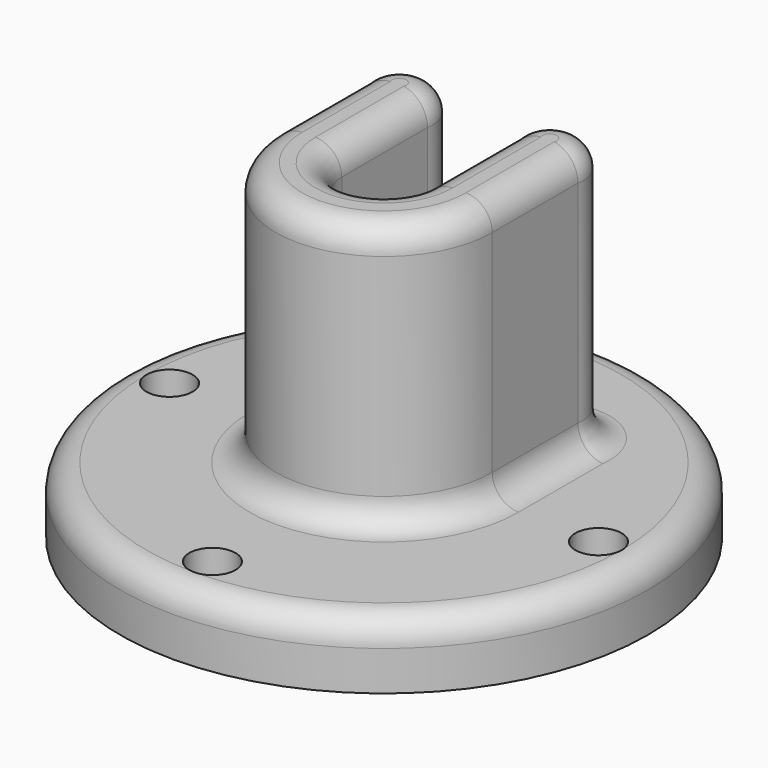
from build123d import *

# Parameters (mm, degrees)
F0_R     = 25.4
F0_R_2   = 2.2225
F1_DEPTH = 6.35
F3_DEPTH = 25.4
F5_R     = 2.54
F6_DEPTH = 25.4


# Not quite as in the source:
# - a feature of the source that left no trace in its solid (it failed there, or was rolled back) is left out


with BuildPart() as f1:
    # F0 (on Top) → F1 (new body)
    with BuildSketch(Plane.XY):
        Circle(F0_R)
        with Locations((0, -20.6375)):
            Circle(F0_R_2, mode=Mode.SUBTRACT)
        with Locations((-20.6375, 0)):
            Circle(F0_R_2, mode=Mode.SUBTRACT)
        with Locations((20.6375, 0)):
            Circle(F0_R_2, mode=Mode.SUBTRACT)
        with BuildLine():
            Line((-4.064, 10.31875), (-4.064, 0))
            ThreePointArc((-4.064, 0), (0, -4.064), (4.064, 0))
            Line((4.064, 0), (4.064, 10.31875))
            ThreePointArc((4.064, 10.31875), (7.239, 14.1114143812), (10.414, 10.31875))
            Line((10.414, 10.31875), (10.414, 0))
            ThreePointArc((10.414, 0), (0, -10.414), (-10.414, 0))
            Line((-10.414, 0), (-10.414, 10.31875))
            ThreePointArc((-10.414, 10.31875), (-7.239, 14.1114143812), (-4.064, 10.31875))
        make_face(mode=Mode.SUBTRACT)
        with Locations((0, 20.6375)):
            Circle(F0_R_2, mode=Mode.SUBTRACT)
        with BuildLine():
            ThreePointArc((4.064, 0), (0, -4.064), (-4.064, 0))
            Line((-4.064, 0), (-4.064, 10.31875))
            ThreePointArc((-4.064, 10.31875), (-7.239, 14.1114143812), (-10.414, 10.31875))
            Line((-10.414, 10.31875), (-10.414, 0))
            ThreePointArc((-10.414, 0), (0, -10.414), (10.414, 0))
            Line((10.414, 0), (10.414, 10.31875))
            ThreePointArc((10.414, 10.31875), (7.239, 14.1114143812), (4.064, 10.31875))
            Line((4.064, 10.31875), (4.064, 0))
        make_face()
        with Locations((0, -20.6375)):
            Circle(F0_R_2)
        with Locations((-20.6375, 0)):
            Circle(F0_R_2)
        with Locations((0, 20.6375)):
            Circle(F0_R_2)
        with Locations((20.6375, 0)):
            Circle(F0_R_2)
    extrude(amount=F1_DEPTH)

    # F2 (on face) → F3 (join)
    with BuildSketch(Plane.XY.offset(6.35)):
        with BuildLine():
            Line((-10.414, 10.31875), (-10.414, 0))
            ThreePointArc((-10.414, 0), (0, -10.414), (10.414, 0))
            Line((10.414, 0), (10.414, 10.31875))
            ThreePointArc((10.414, 10.31875), (7.239, 14.1114143812), (4.064, 10.31875))
            Line((4.064, 10.31875), (4.064, 0))
            ThreePointArc((4.064, 0), (0, -4.064), (-4.064, 0))
            Line((-4.064, 0), (-4.064, 10.31875))
            ThreePointArc((-4.064, 10.31875), (-7.239, 14.1114143812), (-10.414, 10.31875))
        make_face()
    extrude(amount=F3_DEPTH)

    # F5
    f5_edges = [f1.edges().sort_by_distance(p)[0] for p in [
        (-4.064, 5.159375, 31.75),
        (-7.239, 14.111414, 31.75),
        (-10.414, 5.159375, 31.75),
        (0, -10.414, 31.75),
        (10.414, 5.159375, 31.75),
        (7.239, 14.111414, 31.75),
        (4.064, 5.159375, 31.75),
        (0, -4.064, 31.75),
        (-25.4, 0, 6.35),
        (-4.064, 5.159375, 6.35),
        (-7.239, 14.111414, 6.35),
        (-10.414, 5.159375, 6.35),
        (0, -10.414, 6.35),
        (10.414, 5.159375, 6.35),
        (7.239, 14.111414, 6.35),
        (4.064, 5.159375, 6.35),
        (0, -4.064, 6.35),
    ]]
    fillet(f5_edges, radius=F5_R)

    # F0 (on Top) → F6 (cut)
    with BuildSketch(Plane.XY):
        with Locations((20.6375, 0)):
            Circle(F0_R_2)
        with Locations((0, 20.6375)):
            Circle(F0_R_2)
        with Locations((-20.6375, 0)):
            Circle(F0_R_2)
        with Locations((0, -20.6375)):
            Circle(F0_R_2)
    extrude(amount=F6_DEPTH, mode=Mode.SUBTRACT)


solid = f1.part
